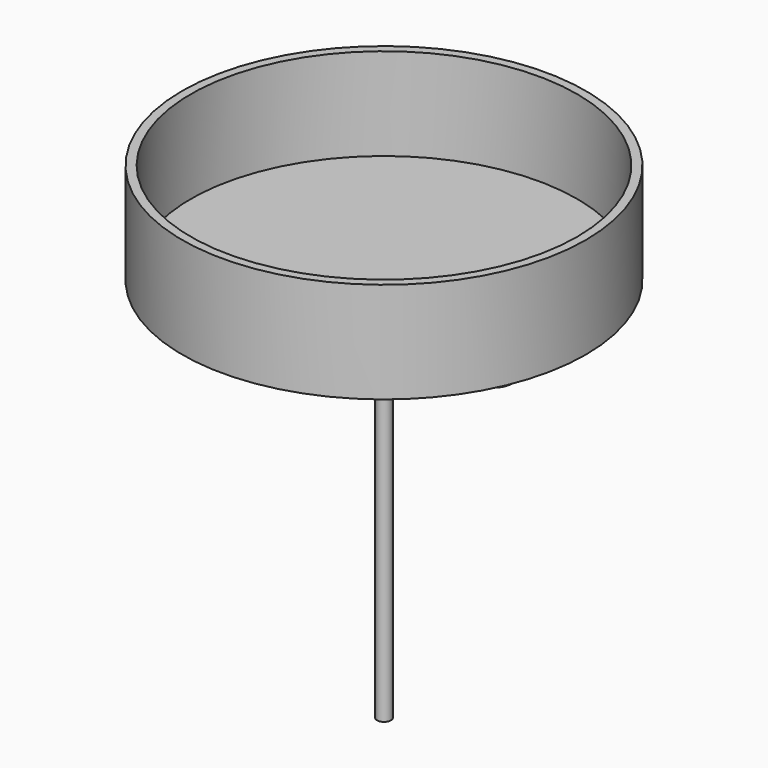
from build123d import *

# Parameters (mm, degrees)
F0_R            = 139.7
F1_DEPTH        = 69.85
F2_T            = -6
F3_R            = 12.7
F3_R_2          = 6.375
F4_DEPTH        = 12
F4_COPIES_COUNT = 5
F6_R            = 4.7625
F7_DEPTH        = 266.7


# Not quite as in the source:
# - a pattern or mirror of a feature is missing from the dataset's text; its kind, count and spacing are read off the source's solid


with BuildPart() as f1:
    # F0 (on Top) → F1 (new body)
    with BuildSketch(Plane.XY):
        Circle(F0_R)
    extrude(amount=F1_DEPTH)

    # F2
    f2_openings = [f1.faces().sort_by_distance(p)[0] for p in [
        (0, 0, 69.85),
    ]]
    offset(amount=F2_T, openings=f2_openings)

    # F3 (on face) → F4 (join)
    with BuildSketch(Plane(origin=(0, 0, 0), x_dir=(1, 0, 0), z_dir=(0, 0, -1))):
        with Locations((0, 107.95)):
            Circle(F3_R)
        with Locations((0, 107.95)):
            Circle(F3_R_2, mode=Mode.SUBTRACT)
    f4 = extrude(amount=F4_DEPTH)

    # F4_copies: F4 ×5 about axis
    f4_copies_axis = Axis((0, 0, 0), (0, 0, 1))
    for i in range(1, F4_COPIES_COUNT):
        add(f4.rotate(f4_copies_axis, i * 360 / F4_COPIES_COUNT))

    # F6 (on face) → F7 (join)
    with BuildSketch(Plane(origin=(0, 0, 0), x_dir=(1, 0, 0), z_dir=(0, 0, -1))):
        Circle(F6_R)
    extrude(amount=F7_DEPTH)


solid = f1.part
